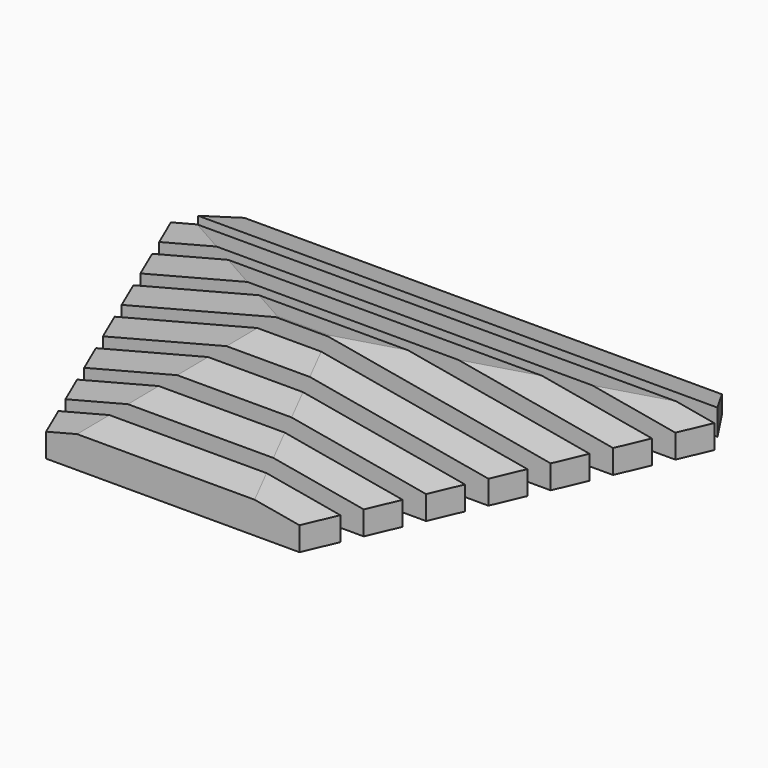
from build123d import *

# Parameters (mm, degrees)
F1_DEPTH = 8
F2_SIZE2 = 18
F2_SIZE  = 5
F3_SIZE2 = 26
F3_SIZE  = 4
F4_SIZE2 = 26
F4_SIZE  = 5
F5_SIZE2 = 23.99999
F5_SIZE  = 5.99999
F6_SIZE  = 8
F8_W     = 49.696596037
F8_H     = 2.4
F9_DEPTH = 36.2


# Not quite as in the source:
# - a fillet or chamfer is up to 0.001 mm smaller than in the source, because OpenCascade refuses the exact size


with BuildPart() as f1:
    # F0 (on Top) → F1 (new body)
    with BuildSketch(Plane.XY):
        Polygon((0, 50), (0, 0), (16, 0), (37.5, 50), align=None)
        Polygon((-16, 0), (0, 0), (0, 50), (-37.5, 50), align=None)
    extrude(amount=F1_DEPTH)

    # F2
    f2_edges = [f1.edges().sort_by_distance(p)[0] for p in [
        (-26.75, 25, 8),
    ]]
    f2_side = f1.faces().sort_by_distance((-26.75, 25, 4))[0]
    chamfer(f2_edges, length=F2_SIZE, length2=F2_SIZE2, reference=f2_side)

    # F3
    f3_edges = [f1.edges().sort_by_distance(p)[0] for p in [
        (9.79678, 0, 8),
    ]]
    f3_side = f1.faces().sort_by_distance((2.240499, 0, 3.447889))[0]
    chamfer(f3_edges, length=F3_SIZE, length2=F3_SIZE2, reference=f3_side)

    # F4
    f4_edges = [f1.edges().sort_by_distance(p)[0] for p in [
        (32.34, 38, 8),
    ]]
    f4_side = f1.faces().sort_by_distance((27.799464, 27.440613, 3.601533))[0]
    chamfer(f4_edges, length=F4_SIZE, length2=F4_SIZE2, reference=f4_side)

    # F5 (size 6 and 24 in the source; OpenCascade refuses exactly that, so slightly less here)
    f5_edges = [f1.edges().sort_by_distance(p)[0] for p in [
        (-4.354124, 50, 8),
    ]]
    f5_side = f1.faces().sort_by_distance((-0.976192, 50, 3.418255))[0]
    chamfer(f5_edges, length=F5_SIZE, length2=F5_SIZE2, reference=f5_side)

    # F6
    f6_edges = [f1.edges().sort_by_distance(p)[0] for p in [
        (-37.5, 50, 1.000005),
        (37.5, 50, 1.000005),
    ]]
    chamfer(f6_edges, length=F6_SIZE)

    # F8 (on offset) → F9 (cut)
    with BuildSketch(Plane.XY.offset(25)):
        with Locations((-24.8482980185, 50.2)):
            Rectangle(F8_W, F8_H)
        with Locations((24.8482980185, 50.2)):
            Rectangle(F8_W, F8_H)
        with Locations((24.8482980185, 43.8)):
            Rectangle(F8_W, F8_H)
        with Locations((24.8482980185, 37.4)):
            Rectangle(F8_W, F8_H)
        with Locations((24.8482980185, 31)):
            Rectangle(F8_W, F8_H)
        with Locations((24.8482980185, 24.6)):
            Rectangle(F8_W, F8_H)
        with Locations((24.8482980185, 18.2)):
            Rectangle(F8_W, F8_H)
        with Locations((24.8482980185, 11.8)):
            Rectangle(F8_W, F8_H)
        with Locations((24.8482980185, 5.4)):
            Rectangle(F8_W, F8_H)
        with Locations((-24.8482980185, 5.4)):
            Rectangle(F8_W, F8_H)
        with Locations((-24.8482980185, 11.8)):
            Rectangle(F8_W, F8_H)
        with Locations((-24.8482980185, 18.2)):
            Rectangle(F8_W, F8_H)
        with Locations((-24.8482980185, 24.6)):
            Rectangle(F8_W, F8_H)
        with Locations((-24.8482980185, 31)):
            Rectangle(F8_W, F8_H)
        with Locations((-24.8482980185, 37.4)):
            Rectangle(F8_W, F8_H)
        with Locations((-24.8482980185, 43.8)):
            Rectangle(F8_W, F8_H)
    extrude(amount=-F9_DEPTH, mode=Mode.SUBTRACT)


solid = f1.part
